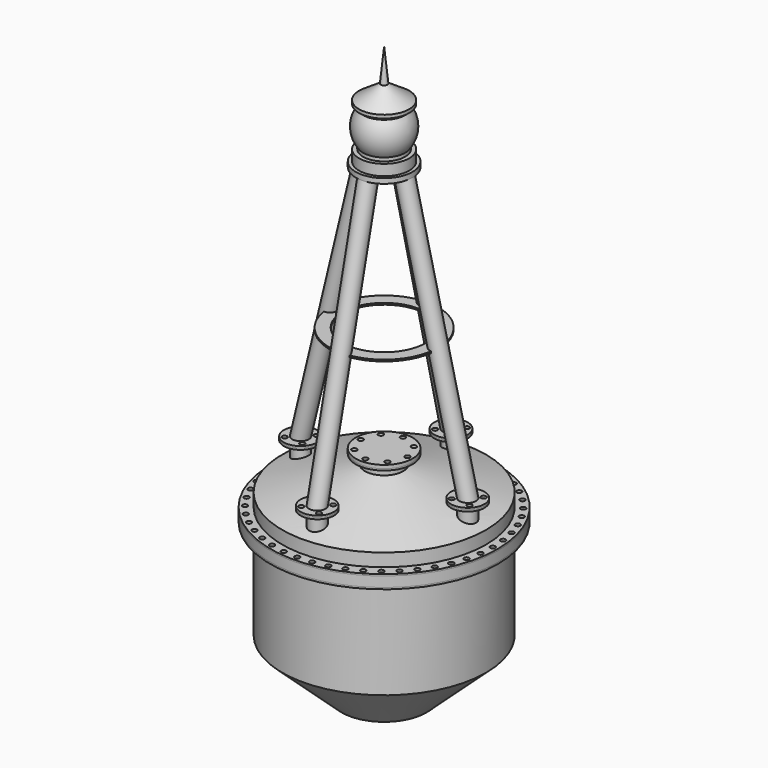
from build123d import *

# Parameters (mm, degrees)
F2_W         = 10
F2_H         = 6
F4_R         = 10
F5_DEPTH     = 3
F6_R         = 17
F7_DEPTH     = 2
F8_R         = 1.5
F9_DEPTH     = 3
F10_R        = 1.5
F1_FACE2_R   = 68
F1_FACE2_R_2 = 61
F11_DEPTH    = 25
F13_R        = 5
F13_R_2      = 4
F15_R        = 10
F15_R_2      = 1.5
F15_R_3      = 4
F16_DEPTH    = 1
F17_R        = 10
F17_R_2      = 1.5
F18_DEPTH    = 1
F19_R        = 5
F24_R        = 5
F27_R        = 5
F30_R        = 5
F33_R        = 17
F33_R_2      = 6
F34_DEPTH    = 3
F36_R        = 25
F37_DEPTH    = 0.5


with BuildPart() as f1:
    # F0 (on Front) → F1 (revolve)
    with BuildSketch(Plane.XZ):
        Polygon((17, 50), (10, 50), (10, 43), (60, 28), (60, 20), (68, 20), (68, 21), (61, 21), (61, 28.7440306509), (11.5, 43.5940306509), (11.5, 49), (17, 49), align=None)
    revolve(axis=Axis((0, 0, 31.8855382502), (0, 0, 1)))


with BuildPart() as f1b:
    # F0 (on Front) → F1, piece 2 (revolve)
    with BuildSketch(Plane.XZ):
        Polygon((68, 13), (68, 14), (60, 14), (60, -46), (25, -78), (0, -78), (0, -79), (25.3882382127, -79), (61, -46.4406749373), (61, 13), align=None)
    revolve(axis=Axis((0, 0, 31.8855382502), (0, 0, 1)))


with BuildPart() as f3:
    # F2 (on Front) → F3 (revolve)
    with BuildSketch(Plane.XZ):
        with Locations((63, 17)):
            Rectangle(F2_W, F2_H)
    revolve(axis=Axis((0, 0, 9.2717269436), (0, 0, -1)))


with BuildPart() as f5:
    # F4 (on face) → F5 (new body)
    with BuildSketch(Plane.XY.offset(50)):
        Circle(F4_R)
    extrude(amount=-F5_DEPTH)

    # F6 (on face) → F7 (join)
    with BuildSketch(Plane.XY.offset(50)):
        Circle(F6_R)
    extrude(amount=F7_DEPTH)

    # F8 (on face) → F9 (cut, through all)
    with BuildSketch(Plane.XY.offset(52)):
        with Locations((0, 14)):
            Circle(F8_R)
        with Locations((-9.8994949366, 9.8994949366)):
            Circle(F8_R)
        with Locations((-14, 0)):
            Circle(F8_R)
        with Locations((-9.8994949366, -9.8994949366)):
            Circle(F8_R)
        with Locations((0, -14)):
            Circle(F8_R)
        with Locations((9.8994949366, -9.8994949366)):
            Circle(F8_R)
        with Locations((14, 0)):
            Circle(F8_R)
        with Locations((9.8994949366, 9.8994949366)):
            Circle(F8_R)
    extrude(amount=-F9_DEPTH, mode=Mode.SUBTRACT)


with BuildPart() as f11_tool:
    # F10 (on face) + F1_face2 (on face) → F11 (new body)
    with BuildSketch(Plane.XY.offset(21)):
        with Locations((-65, 0)):
            Circle(F10_R)
        with Locations((-64.4439159893, -8.4842024943)):
            Circle(F10_R)
        with Locations((-62.7851787088, -16.8232379317)):
            Circle(F10_R)
        with Locations((-60.0521696132, -24.8744231037)):
            Circle(F10_R)
        with Locations((-56.291651246, -32.5)):
            Circle(F10_R)
        with Locations((-51.5679671189, -39.5694928856)):
            Circle(F10_R)
        with Locations((-45.9619407771, -45.9619407771)):
            Circle(F10_R)
        with Locations((-39.5694928856, -51.5679671189)):
            Circle(F10_R)
        with Locations((-32.5, -56.291651246)):
            Circle(F10_R)
        with Locations((-24.8744231037, -60.0521696132)):
            Circle(F10_R)
        with Locations((-16.8232379317, -62.7851787088)):
            Circle(F10_R)
        with Locations((-8.4842024943, -64.4439159893)):
            Circle(F10_R)
        with Locations((0, -65)):
            Circle(F10_R)
        with Locations((8.4842024943, -64.4439159893)):
            Circle(F10_R)
        with Locations((16.8232379317, -62.7851787088)):
            Circle(F10_R)
        with Locations((24.8744231037, -60.0521696132)):
            Circle(F10_R)
        with Locations((32.5, -56.291651246)):
            Circle(F10_R)
        with Locations((39.5694928856, -51.5679671189)):
            Circle(F10_R)
        with Locations((45.9619407771, -45.9619407771)):
            Circle(F10_R)
        with Locations((51.5679671189, -39.5694928856)):
            Circle(F10_R)
        with Locations((56.291651246, -32.5)):
            Circle(F10_R)
        with Locations((60.0521696132, -24.8744231037)):
            Circle(F10_R)
        with Locations((62.7851787088, -16.8232379317)):
            Circle(F10_R)
        with Locations((64.4439159893, -8.4842024943)):
            Circle(F10_R)
        with Locations((65, 0)):
            Circle(F10_R)
        with Locations((64.4439159893, 8.4842024943)):
            Circle(F10_R)
        with Locations((62.7851787088, 16.8232379317)):
            Circle(F10_R)
        with Locations((60.0521696132, 24.8744231037)):
            Circle(F10_R)
        with Locations((56.291651246, 32.5)):
            Circle(F10_R)
        with Locations((51.5679671189, 39.5694928856)):
            Circle(F10_R)
        with Locations((45.9619407771, 45.9619407771)):
            Circle(F10_R)
        with Locations((39.5694928856, 51.5679671189)):
            Circle(F10_R)
        with Locations((32.5, 56.291651246)):
            Circle(F10_R)
        with Locations((24.8744231037, 60.0521696132)):
            Circle(F10_R)
        with Locations((16.8232379317, 62.7851787088)):
            Circle(F10_R)
        with Locations((8.4842024943, 64.4439159893)):
            Circle(F10_R)
        with Locations((0, 65)):
            Circle(F10_R)
        with Locations((-8.4842024943, 64.4439159893)):
            Circle(F10_R)
        with Locations((-16.8232379317, 62.7851787088)):
            Circle(F10_R)
        with Locations((-24.8744231037, 60.0521696132)):
            Circle(F10_R)
        with Locations((-32.5, 56.291651246)):
            Circle(F10_R)
        with Locations((-39.5694928856, 51.5679671189)):
            Circle(F10_R)
        with Locations((-45.9619407771, 45.9619407771)):
            Circle(F10_R)
        with Locations((-51.5679671189, 39.5694928856)):
            Circle(F10_R)
        with Locations((-56.291651246, 32.5)):
            Circle(F10_R)
        with Locations((-60.0521696132, 24.8744231037)):
            Circle(F10_R)
        with Locations((-62.7851787088, 16.8232379317)):
            Circle(F10_R)
        with Locations((-64.4439159893, 8.4842024943)):
            Circle(F10_R)
    with BuildSketch(Plane(origin=(0, 0, 13), x_dir=(1, 0, 0), z_dir=(0, 0, -1))):
        Circle(F1_FACE2_R)
        Circle(F1_FACE2_R_2, mode=Mode.SUBTRACT)
    extrude(amount=-F11_DEPTH, dir=(0, 0, 1))


with BuildPart() as f1_1:
    add(f1.part)

    # F11: cut by f11_tool
    add(f11_tool.part, mode=Mode.SUBTRACT)

    # F13 (on offset) → F14 (join, up to the next surface of F1)
    with BuildSketch(Plane.XY.offset(40)):
        with Locations((0, 50)):
            Circle(F13_R)
        with Locations((0, 50)):
            Circle(F13_R_2, mode=Mode.SUBTRACT)
        with Locations((-50, 0)):
            Circle(F13_R)
        with Locations((-50, 0)):
            Circle(F13_R_2, mode=Mode.SUBTRACT)
        with Locations((0, -50)):
            Circle(F13_R)
        with Locations((0, -50)):
            Circle(F13_R_2, mode=Mode.SUBTRACT)
        with Locations((50, 0)):
            Circle(F13_R)
        with Locations((50, 0)):
            Circle(F13_R_2, mode=Mode.SUBTRACT)
    extrude(until=Until.NEXT, dir=(0, 0, -1))

    # F15 (on offset) → F16 (join)
    with BuildSketch(Plane.XY.offset(40)):
        with Locations((0, 50)):
            Circle(F15_R)
        with Locations((-5.3033008589, 44.6966991411)):
            Circle(F15_R_2, mode=Mode.SUBTRACT)
        with Locations((-5.3033008589, 55.3033008589)):
            Circle(F15_R_2, mode=Mode.SUBTRACT)
        with Locations((5.3033008589, 44.6966991411)):
            Circle(F15_R_2, mode=Mode.SUBTRACT)
        with Locations((0, 50)):
            Circle(F15_R_3, mode=Mode.SUBTRACT)
        with Locations((5.3033008589, 55.3033008589)):
            Circle(F15_R_2, mode=Mode.SUBTRACT)
        with Locations((-50, 0)):
            Circle(F15_R)
        with Locations((-55.3033008589, -5.3033008589)):
            Circle(F15_R_2, mode=Mode.SUBTRACT)
        with Locations((-44.6966991411, -5.3033008589)):
            Circle(F15_R_2, mode=Mode.SUBTRACT)
        with Locations((-55.3033008589, 5.3033008589)):
            Circle(F15_R_2, mode=Mode.SUBTRACT)
        with Locations((-44.6966991411, 5.3033008589)):
            Circle(F15_R_2, mode=Mode.SUBTRACT)
        with Locations((0, -50)):
            Circle(F15_R)
        with Locations((-5.3033008589, -55.3033008589)):
            Circle(F15_R_2, mode=Mode.SUBTRACT)
        with Locations((-5.3033008589, -44.6966991411)):
            Circle(F15_R_2, mode=Mode.SUBTRACT)
        with Locations((5.3033008589, -55.3033008589)):
            Circle(F15_R_2, mode=Mode.SUBTRACT)
        with Locations((5.3033008589, -44.6966991411)):
            Circle(F15_R_2, mode=Mode.SUBTRACT)
        with Locations((50, 0)):
            Circle(F15_R)
        with Locations((44.6966991411, -5.3033008589)):
            Circle(F15_R_2, mode=Mode.SUBTRACT)
        with Locations((55.3033008589, -5.3033008589)):
            Circle(F15_R_2, mode=Mode.SUBTRACT)
        with Locations((44.6966991411, 5.3033008589)):
            Circle(F15_R_2, mode=Mode.SUBTRACT)
        with Locations((55.3033008589, 5.3033008589)):
            Circle(F15_R_2, mode=Mode.SUBTRACT)
        with Locations((0, 50)):
            Circle(F15_R_3)
    extrude(amount=F16_DEPTH)


with BuildPart() as f1b_1:
    add(f1b.part)

    # F11: cut by f11_tool
    add(f11_tool.part, mode=Mode.SUBTRACT)


with BuildPart() as f3_1:
    add(f3.part)

    # F11: cut by f11_tool
    add(f11_tool.part, mode=Mode.SUBTRACT)


with BuildPart() as f18:
    # F17 (on face) → F18 (new body)
    with BuildSketch(Plane.XY.offset(41)):
        with Locations((0, 50)):
            Circle(F17_R)
        with Locations((-5.3033008589, 44.6966991411)):
            Circle(F17_R_2, mode=Mode.SUBTRACT)
        with Locations((-5.3033008589, 55.3033008589)):
            Circle(F17_R_2, mode=Mode.SUBTRACT)
        with Locations((5.3033008589, 44.6966991411)):
            Circle(F17_R_2, mode=Mode.SUBTRACT)
        with Locations((5.3033008589, 55.3033008589)):
            Circle(F17_R_2, mode=Mode.SUBTRACT)
    extrude(amount=F18_DEPTH)

    # F29: sweep along a path in F28
    with BuildLine(Plane.YZ) as f29_path:
        Line((12, 200), (50, 42))
    # F27 (on face) → F29 (sweep)
    with BuildSketch(Plane.XY.offset(42)):
        with Locations((0, 50)):
            Circle(F27_R)
    sweep(path=f29_path.line)


with BuildPart() as f18b:
    # F17 (on face) → F18, piece 2 (new body)
    with BuildSketch(Plane.XY.offset(41)):
        with Locations((-50, 0)):
            Circle(F17_R)
        with Locations((-55.3033008589, -5.3033008589)):
            Circle(F17_R_2, mode=Mode.SUBTRACT)
        with Locations((-44.6966991411, -5.3033008589)):
            Circle(F17_R_2, mode=Mode.SUBTRACT)
        with Locations((-55.3033008589, 5.3033008589)):
            Circle(F17_R_2, mode=Mode.SUBTRACT)
        with Locations((-44.6966991411, 5.3033008589)):
            Circle(F17_R_2, mode=Mode.SUBTRACT)
    extrude(amount=F18_DEPTH)

    # F23: sweep along a path in F22
    with BuildLine(Plane.XZ) as f23_path:
        Line((-50, 42), (-12, 200))
    # F19 (on face) → F23 (sweep)
    with BuildSketch(Plane.XY.offset(42)):
        with Locations((-50, 0)):
            Circle(F19_R)
    sweep(path=f23_path.line)


with BuildPart() as f18c:
    # F17 (on face) → F18, piece 3 (new body)
    with BuildSketch(Plane.XY.offset(41)):
        with Locations((50, 0)):
            Circle(F17_R)
        with Locations((44.6966991411, -5.3033008589)):
            Circle(F17_R_2, mode=Mode.SUBTRACT)
        with Locations((55.3033008589, -5.3033008589)):
            Circle(F17_R_2, mode=Mode.SUBTRACT)
        with Locations((44.6966991411, 5.3033008589)):
            Circle(F17_R_2, mode=Mode.SUBTRACT)
        with Locations((55.3033008589, 5.3033008589)):
            Circle(F17_R_2, mode=Mode.SUBTRACT)
    extrude(amount=F18_DEPTH)

    # F26: sweep along a path in F25
    with BuildLine(Plane.XZ) as f26_path:
        Line((50, 42), (12, 200))
    # F24 (on face) → F26 (sweep)
    with BuildSketch(Plane.XY.offset(42)):
        with Locations((50, 0)):
            Circle(F24_R)
    sweep(path=f26_path.line)


with BuildPart() as f18d:
    # F17 (on face) → F18, piece 4 (new body)
    with BuildSketch(Plane.XY.offset(41)):
        with Locations((0, -50)):
            Circle(F17_R)
        with Locations((-5.3033008589, -55.3033008589)):
            Circle(F17_R_2, mode=Mode.SUBTRACT)
        with Locations((-5.3033008589, -44.6966991411)):
            Circle(F17_R_2, mode=Mode.SUBTRACT)
        with Locations((5.3033008589, -55.3033008589)):
            Circle(F17_R_2, mode=Mode.SUBTRACT)
        with Locations((5.3033008589, -44.6966991411)):
            Circle(F17_R_2, mode=Mode.SUBTRACT)
    extrude(amount=F18_DEPTH)

    # F32: sweep along a path in F31
    with BuildLine(Plane.YZ) as f32_path:
        Line((-12, 200), (-50, 42))
    # F30 (on face) → F32 (sweep)
    with BuildSketch(Plane.XY.offset(42)):
        with Locations((0, -50)):
            Circle(F30_R)
    sweep(path=f32_path.line)


with BuildPart() as f34:
    # F33 (on offset) → F34 (new body)
    with BuildSketch(Plane.XY.offset(200)):
        Circle(F33_R)
        Circle(F33_R_2, mode=Mode.SUBTRACT)
    extrude(amount=F34_DEPTH)


with BuildPart() as f37:
    # F36 (on offset) → F37 (new body, symmetric)
    with BuildSketch(Plane.XY.offset(115)):
        with BuildLine():
            ThreePointArc((-32.1111422115, 5.0124391139), (-27.4725, 0), (-32.1111422115, -5.0124391139))
            ThreePointArc((-32.1111422115, -5.0124391139), (-22.9809703886, -22.9809703886), (-5.0124391139, -32.1111422115))
            ThreePointArc((-5.0124391139, -32.1111422115), (0, -27.4725), (5.0124391139, -32.1111422115))
            ThreePointArc((5.0124391139, -32.1111422115), (22.9809703886, -22.9809703886), (32.1111422115, -5.0124391139))
            ThreePointArc((32.1111422115, -5.0124391139), (27.4725, 0), (32.1111422115, 5.0124391139))
            ThreePointArc((32.1111422115, 5.0124391139), (22.9809703886, 22.9809703886), (5.0124391139, 32.1111422115))
            ThreePointArc((5.0124391139, 32.1111422115), (0, 27.4725), (-5.0124391139, 32.1111422115))
            ThreePointArc((-5.0124391139, 32.1111422115), (-22.9809703886, 22.9809703886), (-32.1111422115, 5.0124391139))
        make_face()
        Circle(F36_R, mode=Mode.SUBTRACT)
    extrude(amount=F37_DEPTH, both=True)


with BuildPart() as f39:
    # F38 (on Front) → F39 (revolve)
    with BuildSketch(Plane.XZ):
        with BuildLine():
            Line((15, 235.3550952894), (0, 238))
            Line((0, 238), (0, 237.4922866941))
            Line((0, 237.4922866941), (12.0595708791, 235.3658589723))
            Line((12.0595708791, 235.3658589723), (12.0595708791, 231.2373892913))
            ThreePointArc((12.0595708791, 231.2373892913), (15.5, 221.5), (12.0595708791, 211.7626107087))
            Line((12.0595708791, 211.7626107087), (12.0595708791, 203.5))
            Line((12.0595708791, 203.5), (0, 203.5))
            Line((0, 203.5), (0, 203))
            Line((0, 203), (15, 203))
            Line((15, 203), (15, 209.5))
            Line((15, 209.5), (12.5595708791, 209.5))
            Line((12.5595708791, 209.5), (12.5595708791, 211.5875240564))
            ThreePointArc((12.5595708791, 211.5875240564), (16, 221.5), (12.5595708791, 231.4124759436))
            Line((12.5595708791, 231.4124759436), (12.5595708791, 233.3550952894))
            Line((12.5595708791, 233.3550952894), (15, 233.3550952894))
            Line((15, 233.3550952894), (15, 235.3550952894))
        make_face()
    revolve(axis=Axis((0, 0, 225.6886957278), (0, 0, 1)))


with BuildPart() as f41:
    # F40 (on Front) → F41 (revolve)
    with BuildSketch(Plane.XZ):
        Polygon((0, 263.7252509594), (0, 238), (15, 235.3550952894), (2, 244), align=None)
    revolve(axis=Axis((0, 0, 250.8626254797), (0, 0, 1)))


solid = Compound([f5.part, f1_1.part, f1b_1.part, f3_1.part, f18.part, f18b.part, f18c.part, f18d.part, f34.part, f37.part, f39.part, f41.part])
